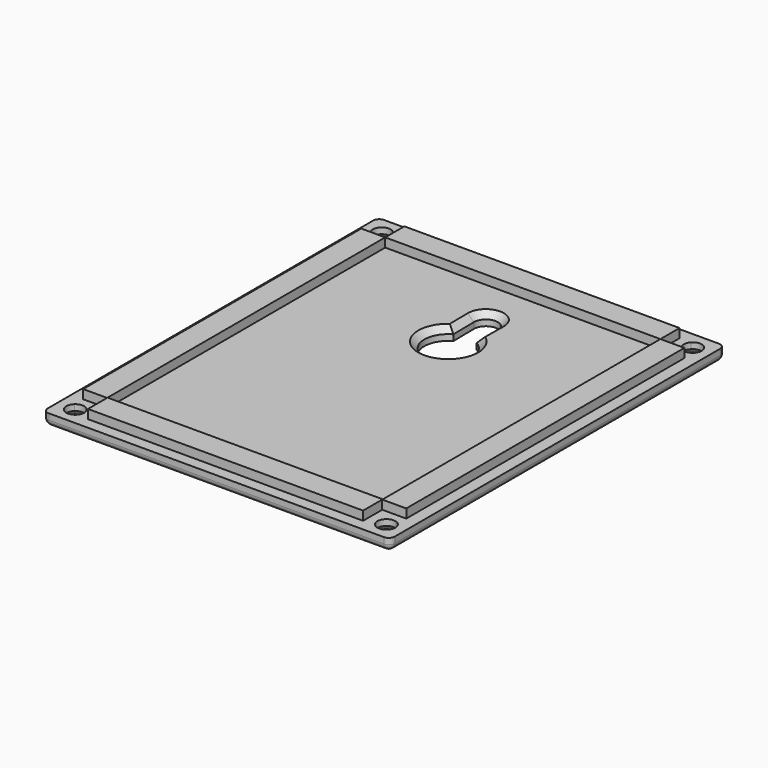
from build123d import *

# Parameters (mm, degrees)
F0_W         = 58
F0_H         = 70
F1_DEPTH     = 2
F2_DEPTH     = 1.5
F3_SIZE      = 1
F4_T1_DEPTH  = 56
F4_T3_DEPTH  = 68
F4_T5_DEPTH  = 3.5
F4_S9_W      = 1
F4_S9_H      = 1
F4_T10_DEPTH = 1
F4_S15_W     = 1
F4_S15_H     = 1
F4_T16_DEPTH = 1
F4_S21_W     = 1
F4_S21_H     = 1
F4_T22_DEPTH = 1
F4_S27_W     = 1
F4_S27_H     = 1
F4_T28_DEPTH = 1
F5_W         = 46
F5_H         = 58
F6_DEPTH     = 1.5
F7_SIZE      = 1


# Not quite as in the source:
# - a fillet or chamfer that OpenCascade refuses, or shapes differently, is made with other operations: its cross-section is extruded or revolved along the edge and cut away or added


with BuildPart() as f1:
    # F0 (on Top) → F1 (new body)
    with BuildSketch(Plane.XY):
        Rectangle(F0_W, F0_H)
        with BuildLine():
            Line((24.9801966052, -33.1000004709), (22.9855267704, -33.1000004709))
            Line((22.9855267704, -33.1000004709), (-23, -33.1000004709))
            Line((-23, -33.1000004709), (-24.9801966052, -33.1000004709))
            ThreePointArc((-24.9801966052, -33.1000004709), (-27.1090614319, -33.009941949), (-27, -30.8819660113))
            Line((-27, -30.8819660113), (-27, -29.1000004709))
            Line((-27, -29.1000004709), (-27, 29))
            Line((-27, 29), (-27, 30.8819660113))
            ThreePointArc((-27, 30.8819660113), (-27.0606601718, 33.0606601718), (-24.8819660113, 33))
            Line((-24.8819660113, 33), (-23, 33))
            Line((-23, 33), (23, 33))
            Line((23, 33), (24.8819660113, 33))
            ThreePointArc((24.8819660113, 33), (26.5352331347, 33.4012585384), (27.5, 32))
            ThreePointArc((27.5, 32), (27.3693063938, 31.3876275643), (27, 30.8819660113))
            Line((27, 30.8819660113), (27, 29))
            Line((27, 29), (27, -29.1000004709))
            Line((27, -29.1000004709), (27, -30.8819660113))
            ThreePointArc((27, -30.8819660113), (27.3693063938, -31.3876275643), (27.5, -32))
            ThreePointArc((27.5, -32), (26.6001228657, -33.374719079), (24.9801966052, -33.1000004709))
        make_face(mode=Mode.SUBTRACT)
        with BuildLine():
            Line((-24.9801966052, -33.1000004709), (-23, -33.1000004709))
            Line((-23, -33.1000004709), (-23, -29.1000004709))
            Line((-23, -29.1000004709), (-27, -29.1000004709))
            Line((-27, -29.1000004709), (-27, -30.8819660113))
            ThreePointArc((-27, -30.8819660113), (-25.3876275643, -30.6306936062), (-24.5, -32))
            ThreePointArc((-24.5, -32), (-24.625280921, -32.6001228657), (-24.9801966052, -33.1000004709))
        make_face()
        Polygon((-23, -33.1000004709), (22.9855267704, -33.1000004709), (22.9855267704, -29.1000004709), (27, -29.1000004709), (27, 29), (23, 29), (23, 33), (-23, 33), (-23, 29), (-27, 29), (-27, -29.1000004709), (-23, -29.1000004709), align=None)
        with BuildLine():
            ThreePointArc((1.9465169508, 16.914761033), (0, 9.4203266352), (-1.9465169508, 16.914761033))
            Line((-1.9465169508, 16.914761033), (-1.9998499612, 21.2685744208))
            ThreePointArc((-1.9998499612, 21.2685744208), (0, 23.2930720299), (1.9998499612, 21.2685744208))
            Line((1.9998499612, 21.2685744208), (1.9465169508, 16.914761033))
        make_face(mode=Mode.SUBTRACT)
        with BuildLine():
            Line((22.9855267704, -29.1000004709), (22.9855267704, -33.1000004709))
            Line((22.9855267704, -33.1000004709), (24.9801966052, -33.1000004709))
            ThreePointArc((24.9801966052, -33.1000004709), (24.8909385681, -30.990058051), (27, -30.8819660113))
            Line((27, -30.8819660113), (27, -29.1000004709))
            Line((27, -29.1000004709), (22.9855267704, -29.1000004709))
        make_face()
        with BuildLine():
            Line((-27, 30.8819660113), (-27, 29))
            Line((-27, 29), (-23, 29))
            Line((-23, 29), (-23, 33))
            Line((-23, 33), (-24.8819660113, 33))
            ThreePointArc((-24.8819660113, 33), (-24.5987414616, 32.5352331347), (-24.5, 32))
            ThreePointArc((-24.5, 32), (-25.3876275643, 30.6306936062), (-27, 30.8819660113))
        make_face()
        with BuildLine():
            Line((23, 29), (27, 29))
            Line((27, 29), (27, 30.8819660113))
            ThreePointArc((27, 30.8819660113), (24.9393398282, 30.9393398282), (24.8819660113, 33))
            Line((24.8819660113, 33), (23, 33))
            Line((23, 33), (23, 29))
        make_face()
    extrude(amount=-F1_DEPTH)

    # F3
    f3_edges = [f1.edges().sort_by_distance(p)[0] for p in [
        (25, 33.118034, -2),
        (-27.118034, 31, -2),
        (27.019803, -30.9, -2),
        (-25, -33.118034, -2),
    ]]
    chamfer(f3_edges, length=F3_SIZE)

    # F4: fillet of radius 1 on 8 edges, made by hand

    # F4_s2 → F4_t1 (cut)
    with BuildSketch(Plane.YZ.offset(-28)):
        with BuildLine():
            ThreePointArc((-34, -2), (-34.7071067812, -1.7071067812), (-35, -1))
            Line((-35, -1), (-35, -2))
            Line((-35, -2), (-34, -2))
        make_face()
        with BuildLine():
            ThreePointArc((34, -2), (34.7071067812, -1.7071067812), (35, -1))
            Line((35, -1), (35, -2))
            Line((35, -2), (34, -2))
        make_face()
    extrude(amount=F4_T1_DEPTH, mode=Mode.SUBTRACT)

    # F4_s4 → F4_t3 (cut)
    with BuildSketch(Plane.XZ.offset(-34)):
        with BuildLine():
            ThreePointArc((-28, -2), (-28.7071067812, -1.7071067812), (-29, -1))
            Line((-29, -1), (-29, -2))
            Line((-29, -2), (-28, -2))
        make_face()
        with BuildLine():
            ThreePointArc((28, -2), (28.7071067812, -1.7071067812), (29, -1))
            Line((29, -1), (29, -2))
            Line((29, -2), (28, -2))
        make_face()
    extrude(amount=F4_T3_DEPTH, mode=Mode.SUBTRACT)

    # F4_s6 → F4_t5 (cut)
    with BuildSketch(Plane.XY.offset(-1)):
        with BuildLine():
            ThreePointArc((-28, 35), (-28.7071067812, 34.7071067812), (-29, 34))
            Line((-29, 34), (-29, 35))
            Line((-29, 35), (-28, 35))
        make_face()
        with BuildLine():
            ThreePointArc((29, 34), (28.7071067812, 34.7071067812), (28, 35))
            Line((28, 35), (29, 35))
            Line((29, 35), (29, 34))
        make_face()
        with BuildLine():
            ThreePointArc((28, -35), (28.7071067812, -34.7071067812), (29, -34))
            Line((29, -34), (29, -35))
            Line((29, -35), (28, -35))
        make_face()
        with BuildLine():
            ThreePointArc((-28, -35), (-28.7071067812, -34.7071067812), (-29, -34))
            Line((-29, -34), (-29, -35))
            Line((-29, -35), (-28, -35))
        make_face()
    extrude(amount=F4_T5_DEPTH, mode=Mode.SUBTRACT)


with BuildPart() as f2:
    # F0 (on Top) → F2 (new body)
    with BuildSketch(Plane.XY):
        Polygon((-23, -33.1000004709), (22.9855267704, -33.1000004709), (22.9855267704, -29.1000004709), (27, -29.1000004709), (27, 29), (23, 29), (23, 33), (-23, 33), (-23, 29), (-27, 29), (-27, -29.1000004709), (-23, -29.1000004709), align=None)
        with BuildLine():
            ThreePointArc((1.9465169508, 16.914761033), (0, 9.4203266352), (-1.9465169508, 16.914761033))
            Line((-1.9465169508, 16.914761033), (-1.9998499612, 21.2685744208))
            ThreePointArc((-1.9998499612, 21.2685744208), (0, 23.2930720299), (1.9998499612, 21.2685744208))
            Line((1.9998499612, 21.2685744208), (1.9465169508, 16.914761033))
        make_face(mode=Mode.SUBTRACT)
    extrude(amount=F2_DEPTH)

    # F5 (on face) → F6 (cut)
    with BuildSketch(Plane.XY.offset(1.5)):
        Rectangle(F5_W, F5_H)
        with BuildLine():
            Line((1.9998499612, 21.2685744208), (1.9465169508, 16.914761033))
            ThreePointArc((1.9465169508, 16.914761033), (0, 9.4203266352), (-1.9465169508, 16.914761033))
            Line((-1.9465169508, 16.914761033), (-1.9998499612, 21.2685744208))
            ThreePointArc((-1.9998499612, 21.2685744208), (0, 23.2930720299), (1.9998499612, 21.2685744208))
        make_face(mode=Mode.SUBTRACT)
    extrude(amount=-F6_DEPTH, mode=Mode.SUBTRACT)


with BuildPart() as f4_tool8:
    # F4_s9 → F4_t10 (new body)
    with BuildSketch(Plane.XY.offset(-1)):
        with Locations((-28.5, -34.5)):
            Rectangle(F4_S9_W, F4_S9_H)
    extrude(amount=-F4_T10_DEPTH)

    # F4_s11 → F4_t12 (revolve, cut)
    with BuildSketch(Plane(origin=(-28, -34, -1), x_dir=(0.7071067812, 0.7071067812, 0), z_dir=(-0.7071067812, 0.7071067812, 0))):
        with BuildLine():
            ThreePointArc((0, -1), (1, 0), (0, 1))
            Line((0, 1), (0, -1))
        make_face()
    revolve(axis=Axis((-28, -34, -1), (0, 0, -1)), mode=Mode.SUBTRACT)


with BuildPart() as f1_1:
    add(f1.part)

    # F4_t7: cut F4_tool8
    add(f4_tool8.part, mode=Mode.SUBTRACT)


with BuildPart() as f4_tool14:
    # F4_s15 → F4_t16 (new body)
    with BuildSketch(Plane.XY.offset(-1)):
        with Locations((28.5, -34.5)):
            Rectangle(F4_S15_W, F4_S15_H)
    extrude(amount=-F4_T16_DEPTH)

    # F4_s17 → F4_t18 (revolve, cut)
    with BuildSketch(Plane(origin=(28, -34, -1), x_dir=(-0.7071067812, 0.7071067812, 0), z_dir=(-0.7071067812, -0.7071067812, 0))):
        with BuildLine():
            ThreePointArc((0, -1), (1, 0), (0, 1))
            Line((0, 1), (0, -1))
        make_face()
    revolve(axis=Axis((28, -34, -1), (0, 0, -1)), mode=Mode.SUBTRACT)


with BuildPart() as f1_2:
    add(f1_1.part)

    # F4_t13: cut F4_tool14
    add(f4_tool14.part, mode=Mode.SUBTRACT)


with BuildPart() as f4_tool20:
    # F4_s21 → F4_t22 (new body)
    with BuildSketch(Plane.XY.offset(-1)):
        with Locations((-28.5, 34.5)):
            Rectangle(F4_S21_W, F4_S21_H)
    extrude(amount=-F4_T22_DEPTH)

    # F4_s23 → F4_t24 (revolve, cut)
    with BuildSketch(Plane(origin=(-28, 34, -1), x_dir=(0.7071067812, -0.7071067812, 0), z_dir=(0.7071067812, 0.7071067812, 0))):
        with BuildLine():
            ThreePointArc((0, -1), (1, 0), (0, 1))
            Line((0, 1), (0, -1))
        make_face()
    revolve(axis=Axis((-28, 34, -1), (0, 0, -1)), mode=Mode.SUBTRACT)


with BuildPart() as f1_3:
    add(f1_2.part)

    # F4_t19: cut F4_tool20
    add(f4_tool20.part, mode=Mode.SUBTRACT)


with BuildPart() as f4_tool26:
    # F4_s27 → F4_t28 (new body)
    with BuildSketch(Plane.XY.offset(-1)):
        with Locations((28.5, 34.5)):
            Rectangle(F4_S27_W, F4_S27_H)
    extrude(amount=-F4_T28_DEPTH)

    # F4_s29 → F4_t30 (revolve, cut)
    with BuildSketch(Plane(origin=(28, 34, -1), x_dir=(-0.7071067812, -0.7071067812, 0), z_dir=(0.7071067812, -0.7071067812, 0))):
        with BuildLine():
            ThreePointArc((0, -1), (1, 0), (0, 1))
            Line((0, 1), (0, -1))
        make_face()
    revolve(axis=Axis((28, 34, -1), (0, 0, -1)), mode=Mode.SUBTRACT)


with BuildPart() as f1_4:
    add(f1_3.part)

    # F4_t25: cut F4_tool26
    add(f4_tool26.part, mode=Mode.SUBTRACT)

    # F7
    f7_edges = [f1_4.edges().sort_by_distance(p)[0] for p in [
        (0, 23.293072, 0),
        (-1.973183, 19.091668, 0),
        (0, 9.420327, 0),
        (1.973183, 19.091668, 0),
    ]]
    chamfer(f7_edges, length=F7_SIZE)


solid = Compound([f2.part, f1_4.part])
